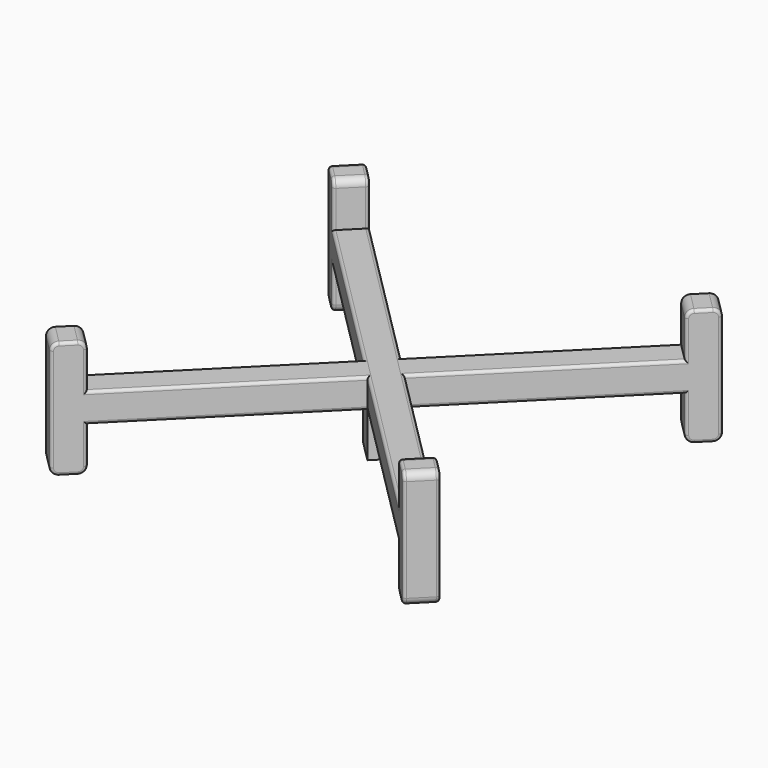
from build123d import *

# Parameters (mm, degrees)
F3_DEPTH      = 12.7
F3_DEPTH_BACK = 12.7
F4_R          = 6.35
F5_R          = 2.54
F7_COUNT      = 2
F7_ANGLE      = 90
F9_DEPTH      = 38.1


with BuildPart() as f3:
    # F2 (on line) → F3 (new body, two sides)
    with BuildSketch(Plane(origin=(0, 0, 0), x_dir=(-0.7071067812, -0.7071067812, 0), z_dir=(-0.7071067812, 0.7071067812, 0))) as f3_sk:
        Polygon((-203.2, 50.8), (-228.6, 50.8), (-228.6, -50.8), (-203.2, -50.8), (-203.2, -12.7), (203.2, -12.7), (203.2, -50.8), (228.6, -50.8), (228.6, 50.8), (203.2, 50.8), (203.2, 12.7), (-203.2, 12.7), align=None)
    extrude(amount=F3_DEPTH)
    extrude(f3_sk.sketch, amount=-F3_DEPTH_BACK)

    # F4
    f4_edges = [f3.edges().sort_by_distance(p)[0] for p in [
        (143.684098, 143.684098, 50.8),
        (-143.684098, -143.684098, 50.8),
        (161.64461, 161.64461, -50.8),
        (-161.64461, -161.64461, -50.8),
        (-161.64461, -161.64461, 50.8),
        (143.684098, 143.684098, -50.8),
        (161.64461, 161.64461, 50.8),
        (-143.684098, -143.684098, -50.8),
    ]]
    fillet(f4_edges, radius=F4_R)

    # F5
    f5_edges = [f3.edges().sort_by_distance(p)[0] for p in [
        (152.664354, 170.624866, 0),
        (-170.624866, -152.664354, 0),
        (-152.664354, -170.624866, 0),
        (-8.980256, 8.980256, 12.7),
        (8.980256, -8.980256, 12.7),
        (-152.664354, -134.703842, 28.575),
        (-8.980256, 8.980256, -12.7),
        (-152.664354, -134.703842, -28.575),
        (134.703842, 152.664354, -28.575),
        (134.703842, 152.664354, 28.575),
        (152.664354, 134.703842, 28.575),
        (157.154482, 157.154482, 50.8),
        (-161.64461, -161.64461, 44.45),
        (-134.703842, -152.664354, -28.575),
        (8.980256, -8.980256, -12.7),
        (-134.703842, -152.664354, 28.575),
        (-136.01897, -153.979482, 48.940128),
        (-148.174226, -148.174226, -50.8),
        (152.664354, 134.703842, -28.575),
        (161.64461, 143.684098, -50.8),
    ]]
    fillet(f5_edges, radius=F5_R)


with BuildPart() as f7_1:
    # F7: instance of F3
    add(f3.part.rotate(Axis((0, 0, -1.0481886566), (0, 0, 1)), 1 * F7_ANGLE / (F7_COUNT - 1)))


with BuildPart() as f9:
    # F8 (on face) → F9 (new body)
    with BuildSketch(Plane(origin=(0, 0, -12.7), x_dir=(1, 0, 0), z_dir=(0, 0, -1))):
        Polygon((17.9605122421, 0), (0, 17.9605122421), (-17.9605122421, 0), (0, -17.9605122421), align=None)
    extrude(amount=F9_DEPTH)


solid = Compound([f3.part, f7_1.part, f9.part])
